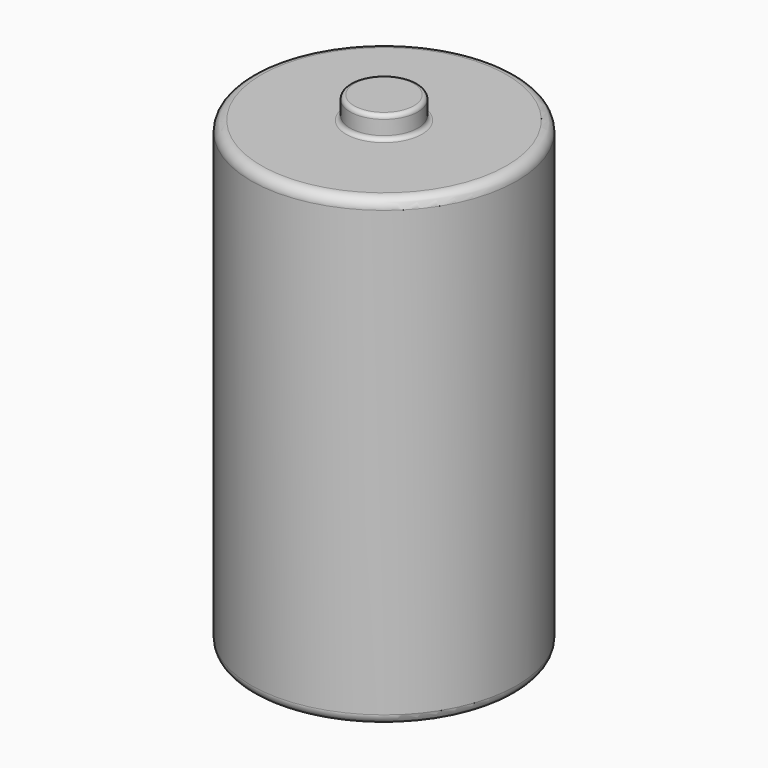
from build123d import *

# Parameters (mm, degrees)
F0_R     = 16.5735
F1_DEPTH = 57.8612
F2_R     = 4.2291
F3_DEPTH = 2.794
F4_R     = 0.508
F5_R     = 1.27
F6_R     = 5.2578
F6_R_2   = 2.9845
F7_DEPTH = 0.508
F9_R     = 0.25399


# Not quite as in the source:
# - a fillet or chamfer that OpenCascade refuses, or shapes differently, is made with other operations: its cross-section is extruded or revolved along the edge and cut away or added
# - a fillet or chamfer is up to 0.001 mm smaller than in the source, because OpenCascade refuses the exact size


with BuildPart() as f1:
    # F0 (on Top) → F1 (new body)
    with BuildSketch(Plane.XY):
        Circle(F0_R)
    extrude(amount=F1_DEPTH)

    # F2 (on face) → F3 (join)
    with BuildSketch(Plane.XY.offset(57.8612)):
        Circle(F2_R)
    extrude(amount=F3_DEPTH)

    # F4
    f4_edges = [f1.edges().sort_by_distance(p)[0] for p in [
        (-4.2291, 0, 60.6552),
        (-4.2291, 0, 57.8612),
    ]]
    fillet(f4_edges, radius=F4_R)

    # F5
    f5_edges = [f1.edges().sort_by_distance(p)[0] for p in [
        (-16.5735, 0, 57.8612),
        (-16.5735, 0, 0),
    ]]
    fillet(f5_edges, radius=F5_R)

    # F6 (on face) → F7 (cut)
    with BuildSketch(Plane(origin=(0, 0, 0), x_dir=(1, 0, 0), z_dir=(0, 0, -1))):
        Circle(F6_R)
        Circle(F6_R_2, mode=Mode.SUBTRACT)
    extrude(amount=-F7_DEPTH, mode=Mode.SUBTRACT)

    # F8: fillet of radius 1.27 on 1 edges, made by hand

    # F8_s1 → F8_t2 (revolve)
    with BuildSketch(Plane.XZ):
        with BuildLine():
            ThreePointArc((4.0005, 0.508), (3.4325387337, 0.3739225326), (2.9845, 0))
            Line((2.9845, 0), (2.9845, 0.508))
            Line((2.9845, 0.508), (4.0005, 0.508))
        make_face()
    revolve(axis=Axis((0, 0, 0.508), (0, 0, -1)))

    # F9 (radius 0.254 in the source; OpenCascade refuses exactly that, so slightly less here)
    f9_edges = [f1.edges().sort_by_distance(p)[0] for p in [
        (-5.2578, 0, 0.508),
        (-5.2578, 0, 0),
    ]]
    fillet(f9_edges, radius=F9_R)


solid = f1.part
